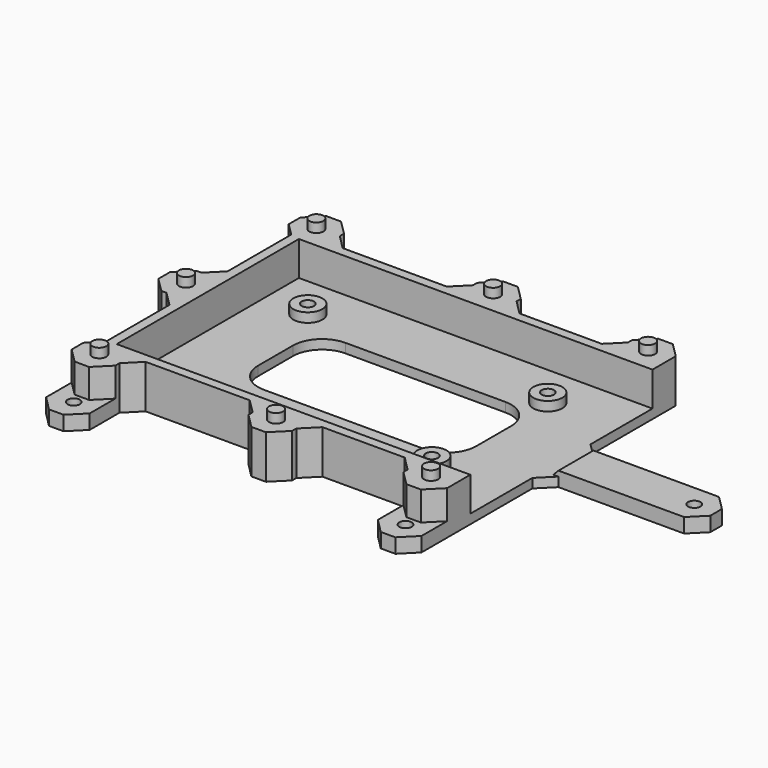
from build123d import *

# Parameters (mm, degrees)
F0_W          = 121.6
F0_H          = 78.3
F0_R          = 2.125
F1_DEPTH      = 3.2
F2_R          = 5
F2_R_2        = 2.125
F3_DEPTH      = 3.2
F5_DEPTH      = 4
F7_DEPTH      = 15
F8_R          = 2.425
F9_DEPTH      = 3.2
F11_W         = 15
F11_H         = 17.8
F11_R         = 2.125
F12_DEPTH     = 5
F13_T1_DEPTH  = 3.2
F13_T3_DEPTH  = 15
F13_T5_DEPTH  = 30.7168298797
F13_T7_DEPTH  = 22.8584149398
F13_T9_DEPTH  = 40.7168298797
F13_T14_DEPTH = 14.6584149398
F13_T19_DEPTH = 14.6584149398
F13_T24_DEPTH = 40.7168298797
F13_T29_DEPTH = 40.7168298797
F13_T34_DEPTH = 40.7168298797


# Not quite as in the source:
# - a fillet or chamfer that OpenCascade refuses, or shapes differently, is made with other operations: its cross-section is extruded or revolved along the edge and cut away or added
# - two fillets or chamfers of one size are made in one step
# - a feature of the source that left no trace in its solid (it failed there, or was rolled back) is left out
# - a feature names something its author has since deleted; it is built from what else it names


with BuildPart() as f1:
    # F0 (on Top) → F1 (new body)
    with BuildSketch(Plane.XY):
        Rectangle(F0_W, F0_H)
        with Locations((35.5, -24.05)):
            Circle(F0_R, mode=Mode.SUBTRACT)
        with BuildLine():
            ThreePointArc((37.5, -7.5), (34.5710678119, -14.5710678119), (27.5, -17.5))
            Line((27.5, -17.5), (-27.5, -17.5))
            ThreePointArc((-27.5, -17.5), (-34.5710678119, -14.5710678119), (-37.5, -7.5))
            Line((-37.5, -7.5), (-37.5, 7.5))
            ThreePointArc((-37.5, 7.5), (-34.5710678119, 14.5710678119), (-27.5, 17.5))
            Line((-27.5, 17.5), (27.5, 17.5))
            ThreePointArc((27.5, 17.5), (34.5710678119, 14.5710678119), (37.5, 7.5))
            Line((37.5, 7.5), (37.5, -7.5))
        make_face(mode=Mode.SUBTRACT)
        with Locations((-45.72, 24.15)):
            Circle(F0_R, mode=Mode.SUBTRACT)
        with Locations((36.8, 24.15)):
            Circle(F0_R, mode=Mode.SUBTRACT)
    extrude(amount=F1_DEPTH)

    # F2 (on face) → F3 (join)
    with BuildSketch(Plane.XY.offset(3.2)):
        with Locations((-45.72, 24.15)):
            Circle(F2_R)
        with Locations((-45.72, 24.15)):
            Circle(F2_R_2, mode=Mode.SUBTRACT)
        with Locations((36.8, 24.15)):
            Circle(F2_R)
        with Locations((36.8, 24.15)):
            Circle(F2_R_2, mode=Mode.SUBTRACT)
        with Locations((35.5, -24.05)):
            Circle(F2_R)
        with Locations((35.5, -24.05)):
            Circle(F2_R_2, mode=Mode.SUBTRACT)
    extrude(amount=F3_DEPTH)

    # F4 (on face) → F5 (cut)
    with BuildSketch(Plane(origin=(0, 0, 0), x_dir=(1, 0, 0), z_dir=(0, 0, -1))):
        Polygon((-44.0312504626, -21.225), (-47.4087495374, -21.225), (-49.0974990748, -24.15), (-47.4087495374, -27.075), (-44.0312504626, -27.075), (-42.3425009252, -24.15), align=None)
        Polygon((38.4887495374, -21.225), (35.1112504626, -21.225), (33.4225009252, -24.15), (35.1112504626, -27.075), (38.4887495374, -27.075), (40.1774990748, -24.15), align=None)
        Polygon((33.8112504626, 21.125), (37.1887495374, 21.125), (38.8774990748, 24.05), (37.1887495374, 26.975), (33.8112504626, 26.975), (32.1225009252, 24.05), align=None)
    extrude(amount=-F5_DEPTH, mode=Mode.SUBTRACT)

    # F6 (on Top) → F7 (join)
    with BuildSketch(Plane.XY):
        Polygon((-60.8, 39.15), (60.8, 39.15), (60.8, 54.15), (45.8, 54.15), (45.8, 42.35), (7.5, 42.35), (7.5, 54.15), (-7.5, 54.15), (-7.5, 42.35), (-53.3, 42.35), (-53.3, 54.15), (-68.3, 54.15), (-68.3, 39.15), (-64, 39.15), (-64, 7.5), (-75.8, 7.5), (-75.8, -7.5), (-64, -7.5), (-64, -39.15), (-68.3, -39.15), (-68.3, -54.15), (-53.3, -54.15), (-53.3, -42.35), (-7.5, -42.35), (-7.5, -54.15), (7.5, -54.15), (7.5, -42.35), (45.8, -42.35), (45.8, -54.15), (60.8, -54.15), (60.8, -39.15), (-60.8, -39.15), align=None)
    extrude(amount=F7_DEPTH)

    # F8 (on face) → F9 (join)
    with BuildSketch(Plane.XY.offset(15)):
        with Locations((53.3, 46.65)):
            Circle(F8_R)
        with Locations((0, 46.65)):
            Circle(F8_R)
        with Locations((-60.8, 46.65)):
            Circle(F8_R)
        with Locations((-68.3, 0)):
            Circle(F8_R)
        with Locations((-60.8, -46.65)):
            Circle(F8_R)
        with Locations((0, -46.65)):
            Circle(F8_R)
        with Locations((53.3, -46.65)):
            Circle(F8_R)
    extrude(amount=F9_DEPTH)

    # F11 (on Top) → F12 (join)
    with BuildSketch(Plane.XY):
        with Locations((53.3, -56.25)):
            Rectangle(F11_W, F11_H)
        with Locations((53.3, -57.65)):
            Circle(F11_R, mode=Mode.SUBTRACT)
        with Locations((-60.8, -56.25)):
            Rectangle(F11_W, F11_H)
        with Locations((-60.8, -57.65)):
            Circle(F11_R, mode=Mode.SUBTRACT)
        Polygon((60.8, -7.5), (64, -7.5), (114, -7.5), (114, 7.5), (64, 7.5), (60.8, 7.5), align=None)
        with Locations((106.5, 0)):
            Circle(F11_R, mode=Mode.SUBTRACT)
    extrude(amount=F12_DEPTH)

    # F13: chamfer of 5 on 37 edges, made by hand

    # F13_s2 → F13_t1 (join)
    with BuildSketch(Plane.XY):
        Polygon((65.8, 7.5), (60.8, 12.5), (60.8, 7.5), align=None)
        Polygon((60.8, -12.5), (65.8, -7.5), (60.8, -7.5), align=None)
    extrude(amount=F13_T1_DEPTH)

    # F13_s4 → F13_t3 (join)
    with BuildSketch(Plane.XY):
        Polygon((45.8, 47.35), (40.8, 42.35), (45.8, 42.35), align=None)
        Polygon((12.5, 42.35), (7.5, 47.35), (7.5, 42.35), align=None)
        Polygon((-7.5, 47.35), (-12.5, 42.35), (-7.5, 42.35), align=None)
        Polygon((-48.3, 42.35), (-53.3, 47.35), (-53.3, 42.35), align=None)
        Polygon((-64, 12.5), (-69, 7.5), (-64, 7.5), align=None)
        Polygon((-69, -7.5), (-64, -12.5), (-64, -7.5), align=None)
        Polygon((-53.3, -47.35), (-48.3, -42.35), (-53.3, -42.35), align=None)
        Polygon((-12.5, -42.35), (-7.5, -47.35), (-7.5, -42.35), align=None)
        Polygon((7.5, -47.35), (12.5, -42.35), (7.5, -42.35), align=None)
        Polygon((40.8, -42.35), (45.8, -47.35), (45.8, -42.35), align=None)
    extrude(amount=F13_T3_DEPTH)

    # F13_s6 → F13_t5 (cut)
    with BuildSketch(Plane.XY.offset(-12.8584149398)):
        Polygon((-68.3, -60.15), (-63.3, -65.15), (-68.3, -65.15), align=None)
        Polygon((-58.3, -65.15), (-53.3, -60.15), (-53.3, -65.15), align=None)
        Polygon((50.8, -65.15), (45.8, -60.15), (45.8, -65.15), align=None)
        Polygon((60.8, -60.15), (55.8, -65.15), (60.8, -65.15), align=None)
        Polygon((114, 2.5), (109, 7.5), (114, 7.5), align=None)
        Polygon((109, -7.5), (114, -2.5), (114, -7.5), align=None)
    extrude(amount=F13_T5_DEPTH, mode=Mode.SUBTRACT)

    # F13_s8 → F13_t7 (cut)
    with BuildSketch(Plane.XY.offset(5)):
        Polygon((60.8, -49.15), (55.8, -54.15), (60.8, -54.15), align=None)
        Polygon((-68.3, -49.15), (-63.3, -54.15), (-68.3, -54.15), align=None)
        Polygon((-53.3, -49.15), (-58.3, -54.15), (-53.3, -54.15), align=None)
        Polygon((50.8, -54.15), (45.8, -49.15), (45.8, -54.15), align=None)
    extrude(amount=F13_T7_DEPTH, mode=Mode.SUBTRACT)

    # F13_s10 → F13_t9 (cut)
    with BuildSketch(Plane.XY.offset(-12.8584149398)):
        Polygon((60.8, 49.15), (55.8, 54.15), (60.8, 54.15), align=None)
        Polygon((50.8, 54.15), (45.8, 49.15), (45.8, 54.15), align=None)
        Polygon((7.5, 49.15), (2.5, 54.15), (7.5, 54.15), align=None)
        Polygon((-2.5, 54.15), (-7.5, 49.15), (-7.5, 54.15), align=None)
        Polygon((-53.3, 49.15), (-58.3, 54.15), (-53.3, 54.15), align=None)
        Polygon((-63.3, 54.15), (-68.3, 49.15), (-68.3, 54.15), align=None)
        Polygon((-70.8, 7.5), (-75.8, 2.5), (-75.8, 7.5), align=None)
        Polygon((-75.8, -2.5), (-70.8, -7.5), (-75.8, -7.5), align=None)
        Polygon((-7.5, -49.15), (-2.5, -54.15), (-7.5, -54.15), align=None)
        Polygon((2.5, -54.15), (7.5, -49.15), (7.5, -54.15), align=None)
    extrude(amount=F13_T9_DEPTH, mode=Mode.SUBTRACT)


with BuildPart() as f13_tool12:
    # F13_s13 → F13_t14 (new body)
    with BuildSketch(Plane.XY.offset(3.2)):
        Polygon((65.8, 7.5), (60.8, 2.5), (60.8, 7.5), align=None)
    extrude(amount=F13_T14_DEPTH)

    split(bisect_by=Plane(origin=(30.4, 0, -30.4), x_dir=(0, 1, 0), z_dir=(-0.7071067812, 0, 0.7071067812)), keep=Keep.TOP)


with BuildPart() as f1_1:
    add(f1.part)

    # F13_t11: cut F13_tool12
    add(f13_tool12.part, mode=Mode.SUBTRACT)


with BuildPart() as f13_tool17:
    # F13_s18 → F13_t19 (new body)
    with BuildSketch(Plane.XY.offset(3.2)):
        Polygon((65.8, -7.5), (60.8, -2.5), (60.8, -7.5), align=None)
    extrude(amount=F13_T19_DEPTH)

    split(bisect_by=Plane(origin=(30.4, 0, -30.4), x_dir=(0, 1, 0), z_dir=(-0.7071067812, 0, 0.7071067812)), keep=Keep.TOP)


with BuildPart() as f1_2:
    add(f1_1.part)

    # F13_t16: cut F13_tool17
    add(f13_tool17.part, mode=Mode.SUBTRACT)


with BuildPart() as f13_tool22:
    # F13_s23 → F13_t24 (new body)
    with BuildSketch(Plane.XZ.offset(-20.3584149398)):
        Polygon((60.8, 0), (65.8, 5), (60.8, 5), align=None)
    extrude(amount=F13_T24_DEPTH)

    split(bisect_by=Plane.XY.offset(3.2), keep=Keep.TOP)


with BuildPart() as f1_3:
    add(f1_2.part)

    # F13_t21: cut F13_tool22
    add(f13_tool22.part, mode=Mode.SUBTRACT)


with BuildPart() as f13_tool27:
    # F13_s28 → F13_t29 (new body)
    with BuildSketch(Plane.XY.offset(-12.8584149398)):
        Polygon((-68.3, 44.15), (-63.3, 39.15), (-68.3, 39.15), align=None)
    extrude(amount=F13_T29_DEPTH)

    split(bisect_by=Plane.YZ.offset(-64), keep=Keep.BOTTOM)


with BuildPart() as f1_4:
    add(f1_3.part)

    # F13_t26: cut F13_tool27
    add(f13_tool27.part, mode=Mode.SUBTRACT)


with BuildPart() as f13_tool32:
    # F13_s33 → F13_t34 (new body)
    with BuildSketch(Plane.XY.offset(-12.8584149398)):
        Polygon((-63.3, -39.15), (-68.3, -44.15), (-68.3, -39.15), align=None)
    extrude(amount=F13_T34_DEPTH)

    split(bisect_by=Plane.YZ.offset(-64), keep=Keep.BOTTOM)


with BuildPart() as f1_5:
    add(f1_4.part)

    # F13_t31: cut F13_tool32
    add(f13_tool32.part, mode=Mode.SUBTRACT)


solid = f1_5.part
